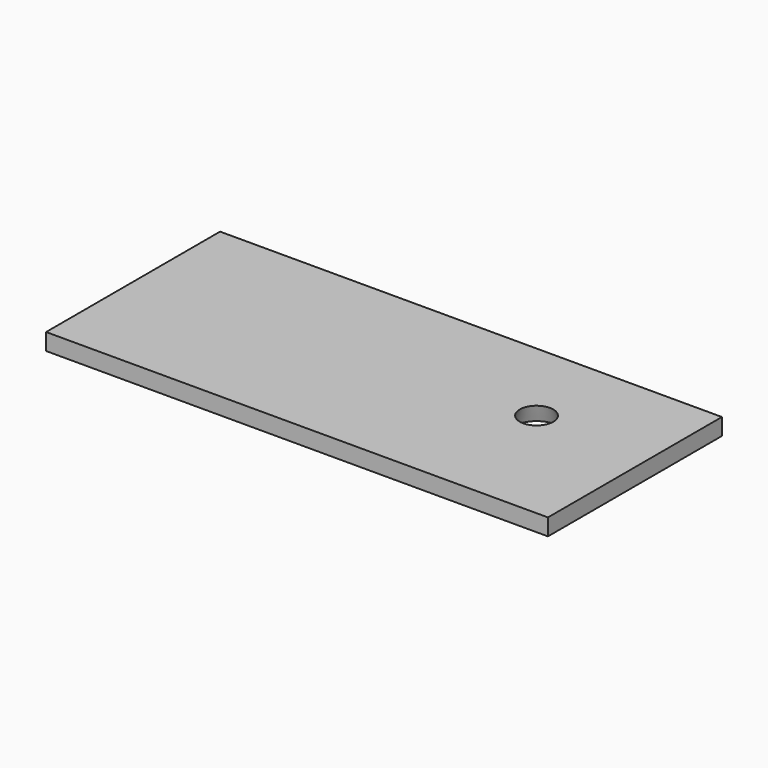
from build123d import *

# Parameters (mm, degrees)
F0_W     = 300
F0_H     = 130
F1_DEPTH = 10
F2_R     = 10
F3_DEPTH = 25
F3_TAPER = -20


with BuildPart() as f1:
    # F0 (on Top) → F1 (new body)
    with BuildSketch(Plane.XY):
        with Locations((40.9527814948, 10.3597547859)):
            Rectangle(F0_W, F0_H)
    extrude(amount=F1_DEPTH)

    # F2 (on face) → F3 (cut)
    with BuildSketch(Plane.XY.offset(10)):
        with Locations((122.5043311715, 22.395953536)):
            Circle(F2_R)
    extrude(amount=-F3_DEPTH, taper=F3_TAPER, mode=Mode.SUBTRACT)


solid = f1.part
